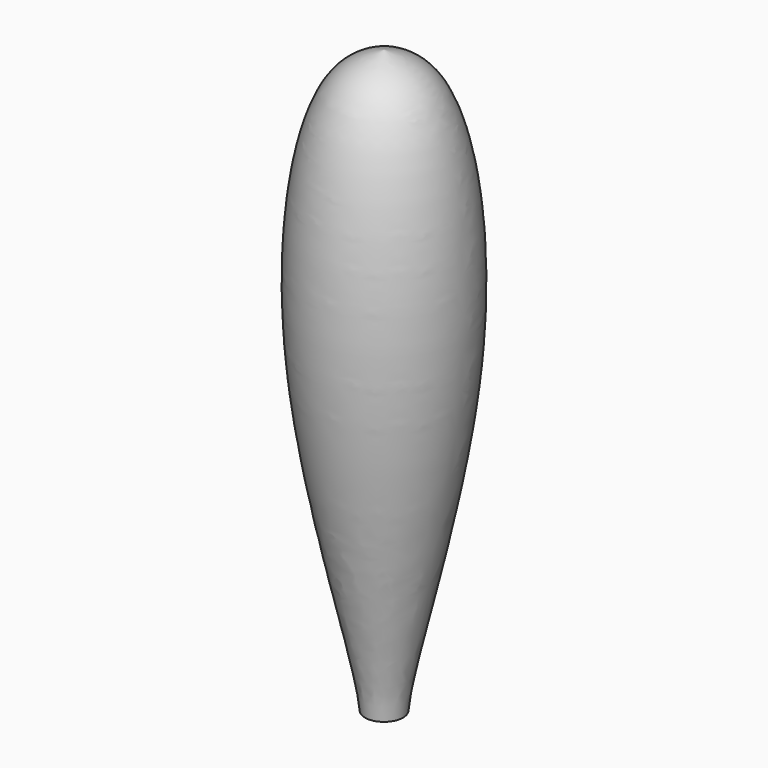
from build123d import *


with BuildPart() as f1:
    # F0 (on Front) → F1 (revolve)
    with BuildSketch(Plane.XZ):
        with BuildLine():
            add(Edge.make_bspline(
                [(0, 0), (1.1635674978, -0.3685194541), (4.8585889027, -1.538786288), (7.1721227943, -20.1214360411), (1.589939134, -38.1407287304), (1.3513215818, -41.2801206112)],
                knots=[0, 0, 0, 0, 0.087553159, 0.2780334752, 0.4852624296, 0.4852624296, 0.4852624296, 0.4852624296], degree=3))
            Line((0, 0), (0, -41.2801206112))
            Line((0, -41.2801206112), (1.3513215818, -41.2801206112))
        make_face()
    revolve(axis=Axis((0, 0, -22.1709161997), (0, 0, -1)))


solid = f1.part
